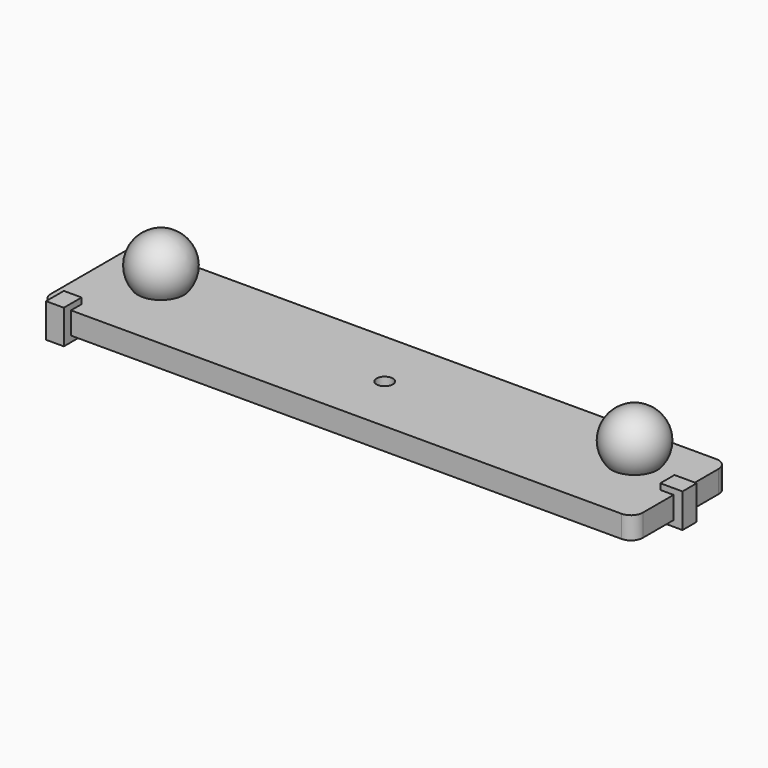
from build123d import *

# Parameters (mm, degrees)
F0_W     = 400
F0_H     = 80
F1_DEPTH = 7.5
F2_R     = 8
F3_W     = 12
F3_H     = 15
F3_W_2   = 15
F3_H_2   = 12
F4_DEPTH = 11.5
F5_R     = 5.5
F6_DEPTH = 25


# Not quite as in the source:
# - a pattern or mirror of a feature is missing from the dataset's text; its kind, count and spacing are read off the source's solid


with BuildPart() as f1:
    # F0 (on Top) → F1 (new body, symmetric)
    with BuildSketch(Plane.XY):
        Rectangle(F0_W, F0_H)
    extrude(amount=F1_DEPTH, both=True)

    # F2
    f2_edges = [f1.edges().sort_by_distance(p)[0] for p in [
        (-200, -40, 0),
        (200, -40, 0),
        (200, 40, 0),
        (-200, 40, 0),
    ]]
    fillet(f2_edges, radius=F2_R)

    # F3 (on Top) → F4 (join, symmetric)
    with BuildSketch(Plane.XY):
        with Locations((-186, -38.5)):
            Rectangle(F3_W, F3_H)
        with Locations((-186, 38.5)):
            Rectangle(F3_W, F3_H)
        with Locations((198.5, 0)):
            Rectangle(F3_W_2, F3_H_2)
    extrude(amount=F4_DEPTH, both=True)

    # F5 (on face) → F6 (cut)
    with BuildSketch(Plane.XY.offset(7.5)):
        Circle(F5_R)
    extrude(amount=-F6_DEPTH, mode=Mode.SUBTRACT)

    # F10 (on plane+point) → F11 (revolve)
    with BuildSketch(Plane.XZ.offset(-11)):
        with BuildLine():
            Line((-160, 40), (-160, 0))
            ThreePointArc((-160, 0), (-140, 20), (-160, 40))
        make_face()
    f11 = revolve(axis=Axis((-160, 11, 20), (0, 0, 1)))

    # F11_copies: F11 across plane
    add(f11.mirror(Plane(origin=(0, 0, 0), x_dir=(0, 0, 1), z_dir=(1, 0, 0))))


solid = f1.part
